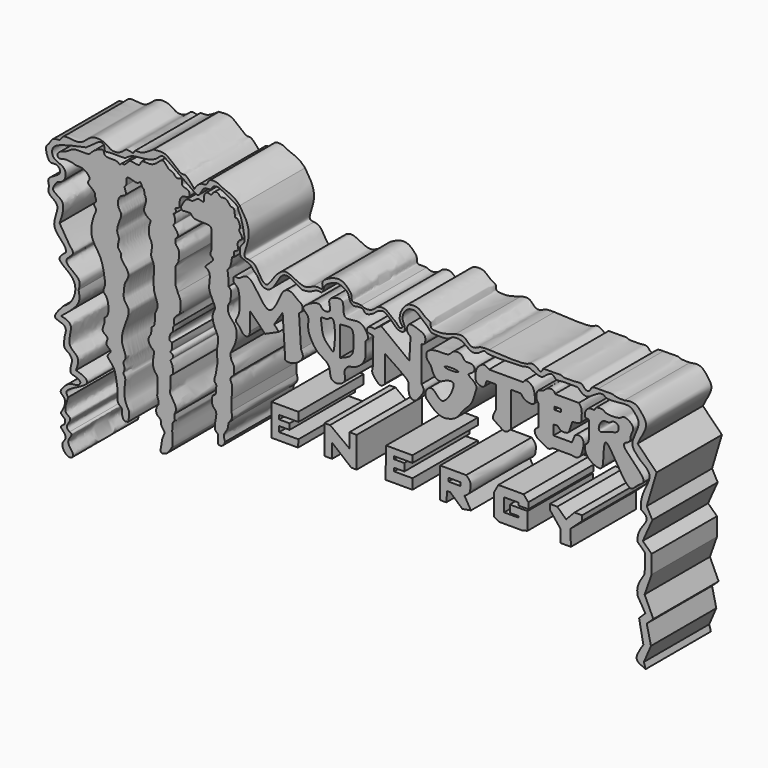
from build123d import *

# Parameters (mm, degrees)
F3_DEPTH = 25
F2_W     = 3.7656910717
F2_H     = 1.0270066559
F2_W_2   = 2.1294355392
F2_H_2   = 0.8966038004


# Not quite as in the source:
# - the program builds the solid bodies; features that only make, move or delete a surface that nothing else refers to are left out


with BuildPart() as f3:
    # F2 (on Front) → F3 (new body)
    with BuildSketch(Plane.XZ):
        Polygon((-21.8279026449, -32.0507697761), (-13.6387161911, -32.0507697761), (-13.5350553319, -29.7702345997), (-19.4437094033, -29.7702345997), (-19.4437094033, -28.1116645783), (-16.230231151, -28.1116645783), (-16.230231151, -26.3494346291), (-19.4437094033, -26.3494346291), (-19.4437094033, -25.1055080444), (-13.5350553319, -25.1055080444), (-13.5350553319, -22.3585031927), (-21.8279026449, -22.3585031927), align=None)
    extrude(amount=F3_DEPTH)


with BuildPart() as f3b:
    # F2 (on Front) → F3, piece 2 (new body)
    with BuildSketch(Plane.XZ):
        Polygon((-3.8289250806, -22.7761287242), (-5.5911550298, -22.8279586881), (-5.5911550298, -31.6909402609), (-3.2069615554, -31.6909402609), (-3.2069615554, -27.3371953517), (2.6498620864, -32.1574136615), (4.3084332719, -32.1574136615), (4.3084332719, -22.7761287242), (2.079728758, -22.7761287242), (2.079728758, -27.1817035973), align=None)
    extrude(amount=F3_DEPTH)


with BuildPart() as f3c:
    # F2 (on Front) → F3, piece 3 (new body)
    with BuildSketch(Plane.XZ):
        Polygon((21.3820878416, -22.7204784751), (13.3220171556, -22.7204784751), (13.1144626066, -32.0258811116), (21.3820878416, -32.0258811116), (21.3820878416, -28.9125498384), (15.7780908048, -28.9125498384), (15.7780908048, -27.909366414), (18.891422078, -27.909366414), (18.891422078, -25.6262551993), (15.7089047134, -25.6262551993), (15.7089047134, -24.7960332781), (21.3820878416, -24.7960332781), align=None)
    extrude(amount=F3_DEPTH)


with BuildPart() as f3d:
    # F2 (on Front) → F3, piece 4 (new body)
    with BuildSketch(Plane.XZ):
        with BuildLine():
            Line((29.8660583794, -32.0507697761), (31.7277424037, -32.0507697761))
            Line((31.7277424037, -32.0507697761), (32.0186279714, -28.9156045765))
            Line((32.0186279714, -28.9156045765), (32.9494699836, -28.9156045765))
            Line((32.9494699836, -28.9156045765), (36.6728305817, -32.2317257524))
            Line((36.6728305817, -32.2317257524), (39.2908193171, -31.7663066089))
            Line((39.2908193171, -31.7663066089), (37.3127833009, -28.450185433))
            add(Edge.make_bspline(
                [(37.8363840282, -22.7204784751), (38.3456048869, -23.1865278474), (39.3238666476, -24.0818530718), (39.1050914631, -25.8334312431), (38.977892404, -27.3696127917), (37.8928678318, -28.0737395457), (37.3127833009, -28.450185433)],
                knots=[0, 0, 0, 0, 0.2644850367, 0.5081009414, 0.7370169838, 1, 1, 1, 1], degree=3))
            Line((37.8363840282, -22.7204784751), (29.8660583794, -22.7204784751))
            Line((29.8660583794, -22.7204784751), (29.8660583794, -32.0507697761))
        make_face()
        with Locations((34.2598091811, -25.7162433118)):
            Rectangle(F2_W, F2_H, mode=Mode.SUBTRACT)
    extrude(amount=F3_DEPTH)


with BuildPart() as f3e:
    # F2 (on Front) → F3, piece 5 (new body)
    with BuildSketch(Plane.XZ):
        Polygon((47.8596165776, -32.0507697761), (55.1240593195, -32.0507697761), (56.6234141588, -31.6276736557), (56.6234141588, -26.305552572), (51.1786416173, -26.305552572), (51.1786416173, -28.5543948412), (53.8787283003, -28.5543948412), (53.8787283003, -28.990233317), (49.4352839887, -28.990233317), (49.4352839887, -24.9151382595), (53.8787283003, -24.9151382595), (53.8787283003, -25.7161445916), (56.8536892533, -25.7161445916), (56.8536892533, -23.8481462002), (55.4007999599, -22.1633397041), (47.6769925559, -22.1633397041), (46.4067310095, -24.4708117098), (46.4067310095, -31.2509573996), align=None)
    extrude(amount=F3_DEPTH)


with BuildPart() as f3f:
    # F2 (on Front) → F3, piece 6 (new body)
    with BuildSketch(Plane.XZ):
        Polygon((66.6389763355, -31.6276736557), (69.8906779289, -31.6276736557), (69.7407498956, -26.8117766827), (73.2039138675, -23.625664413), (73.3251263795, -22.0095198601), (70.9874853492, -22.0095198601), (68.4235452277, -24.7108214691), (65.7234713435, -22.1480466425), (63.4608715773, -22.1480466425), (63.4608715773, -23.7180143595), (66.6389763355, -27.7352873236), align=None)
    extrude(amount=F3_DEPTH)


with BuildPart() as f3g:
    # F2 (on Front) → F3, piece 7 (new body)
    with BuildSketch(Plane.XZ):
        with BuildLine():
            add(Edge.make_bspline(
                [(3.503452288, -4.7838860191), (2.8113226503, -5.0136695081), (1.7830241675, -4.8630734081), (0.0911722194, -6.7811448987), (1.3671495093, -9.3955288011), (-1.4418505197, -11.2815872593), (-4.1217897443, -10.3505317517), (-3.5555284745, -6.4965573266), (-7.1381809371, -4.9981730676), (-9.1052398705, -2.8089888848), (-11.0325887604, 0.9634765262), (-10.0411178915, 4.3471198689), (-11.9148876299, 5.5223323903), (-12.4373031281, 6.7516798684), (-6.8099838065, 9.8665488087), (-6.462441494, 7.1877744687), (-2.9120184289, 7.5155698662), (-5.0031559191, 11.1051679105), (-1.8479274649, 12.3233814583), (0.6824877872, 12.1855257293), (-0.2774898152, 7.0730316824), (3.5047921516, 7.8935101918), (6.0050121897, 7.9486113123), (7.6235614634, 5.625519934), (7.9974005866, 3.995709803), (6.4584911773, 3.5935713271), (8.0066750098, -1.999760349), (4.6370015267, -4.4075534873), (3.503452288, -4.7838860191)],
                knots=[0, 0, 0, 0, 0.0315220967, 0.0654446519, 0.1026152705, 0.1419423819, 0.1771472788, 0.2195443707, 0.263519259, 0.3050564981, 0.3533625845, 0.3957388119, 0.4280430375, 0.4505910626, 0.5046572349, 0.5359398579, 0.5707371212, 0.6103314602, 0.6494294844, 0.6822119863, 0.7277784762, 0.7674991504, 0.8053447517, 0.8441561314, 0.8719949007, 0.8952996773, 0.9483740519, 1, 1, 1, 1], degree=3))
        make_face()
        with BuildLine():
            add(Edge.make_bspline(
                [(-3.3008460887, -2.4911721703), (-3.7924419075, -2.0137396744), (-5.5897346622, -0.5109165894), (-6.3523235923, 1.7697391653), (-6.4166270756, 3.9327068913), (-6.9610982752, 5.752738943), (-4.5225481233, 5.2057664601), (-4.252961633, 5.9994852498), (-1.8495900551, 7.0522733141), (-2.4371710556, -3.4390093796), (-3.1018362507, -2.6844483537), (-3.3008460887, -2.4911721703)],
                knots=[0, 0, 0, 0, 0.1325905556, 0.2546628881, 0.3725255143, 0.4599015989, 0.5640922214, 0.6328553126, 0.7173438444, 0.9463241468, 1, 1, 1, 1], degree=3))
        make_face(mode=Mode.SUBTRACT)
        with BuildLine():
            Line((-0.8801673539, -3.7418559659), (-0.8801673539, 5.3356890567))
            add(Edge.make_bspline(
                [(-0.8801673539, -3.7418559659), (0.1051218784, -3.3629410883), (1.8893722855, -2.6767679297), (3.4229442665, -1.1878230291), (3.2897460639, 2.5173382681), (3.3267032878, 4.3339201727), (2.7130035187, 5.6249956516), (0.9045163806, 5.5591126678), (-0.2714937046, 5.4118885883), (-0.8801673539, 5.3356890567)],
                knots=[0, 0, 0, 0, 0.1705659116, 0.3088761019, 0.495841013, 0.6324582839, 0.7383649585, 0.8645841924, 1, 1, 1, 1], degree=3))
        make_face(mode=Mode.SUBTRACT)
    extrude(amount=F3_DEPTH)


with BuildPart() as f3h:
    # F2 (on Front) → F3, piece 8 (new body)
    with BuildSketch(Plane.XZ):
        with BuildLine():
            Line((13.0070131272, -6.1348984018), (13.0070131272, 1.909989398))
            add(Edge.make_bspline(
                [(24.1350065917, -2.6675420813), (24.4988556117, -3.1186405426), (25.3127079876, -4.1276512428), (23.650589719, -6.2059967045), (22.2456584652, -8.257711553), (19.9145445459, -7.0406724044), (20.3702129266, -3.7004981152), (19.5456257752, -2.444477126), (15.7190605129, 0.103869325), (13.0070131272, 1.909989398)],
                knots=[0, 0, 0, 0, 0.1108514285, 0.2479509179, 0.379166634, 0.4977873803, 0.650360402, 0.752195744, 1, 1, 1, 1], degree=3))
            Line((24.1350065917, -2.6675420813), (24.1350065917, 8.1594744697))
            add(Edge.make_bspline(
                [(20.7801572978, 9.0236030519), (20.3457138528, 9.3864533714), (19.4836634842, 10.1064440978), (19.8580530262, 11.8427016223), (20.7640873111, 12.7051879525), (23.6254897157, 11.6752187346), (25.5643978554, 10.8490187459), (25.2435917704, 8.2790753792), (24.4553801465, 8.1940383167), (24.1350065917, 8.1594744697)],
                knots=[0, 0, 0, 0, 0.1400032029, 0.2778032769, 0.3898219931, 0.5785225018, 0.7357644761, 0.8925998151, 1, 1, 1, 1], degree=3))
            Line((20.7801572978, 9.0236030519), (20.4243399203, 2.4155643769))
            Line((20.4243399203, 2.4155643769), (11.7830587551, 9.0236030519))
            Line((11.7830587551, 9.0236030519), (9.7907502204, 7.5596827082))
            add(Edge.make_bspline(
                [(9.319582954, 4.8124021851), (9.3803734347, 5.0462029175), (9.5213533732, 5.5884130216), (8.2738494629, 5.8541952014), (7.31455102, 5.9431960106), (7.6227500043, 7.9209294321), (9.0216714014, 7.6878317747), (9.7907502204, 7.5596827082)],
                knots=[0, 0, 0, 0, 0.1505740167, 0.3491980219, 0.518685682, 0.7353899597, 1, 1, 1, 1], degree=3))
            Line((9.319582954, 4.8124021851), (9.319582954, -2.5581021328))
            add(Edge.make_bspline(
                [(13.0070131272, -6.1348984018), (12.6049051159, -6.6177685747), (11.7230780125, -7.6767079492), (9.7804141481, -5.6927668504), (8.8350286003, -4.3052662439), (9.1578579839, -3.1412360196), (9.319582954, -2.5581021328)],
                knots=[0, 0, 0, 0, 0.2356288847, 0.5167366256, 0.7579038379, 1, 1, 1, 1], degree=3))
        make_face()
    extrude(amount=F3_DEPTH)


with BuildPart() as f3i:
    # F2 (on Front) → F3, piece 9 (new body)
    with BuildSketch(Plane.XZ):
        with BuildLine():
            add(Edge.make_bspline(
                [(25.5756434053, -6.0040308163), (25.4061184127, -5.3832063219), (25.0512461325, -4.0836138516), (27.7019975714, -1.5243889893), (30.5978060983, -8.0140858299), (35.5163682682, 1.9393601204), (32.6292719516, 1.0476557915), (31.5465591848, 0.7132507162)],
                knots=[0, 0, 0, 0, 0.1540710504, 0.3225220314, 0.5423303079, 0.8283656781, 1, 1, 1, 1], degree=3))
            add(Edge.make_bspline(
                [(31.5465591848, 0.7132507162), (30.7752444483, 0.2979041147), (29.2896538825, -0.502074109), (27.5616896872, 1.2528426912), (27.2311493936, 3.3454250283), (25.4632454929, 4.7198831161), (25.630185434, 6.9245563777), (27.5651484443, 7.7095666937), (29.4398172278, 7.9487657515), (32.7819511773, 7.6664383296), (33.6271863146, 9.6029162043), (36.6279698804, 9.746479837), (37.2599515094, 7.3287532722), (40.1594276723, 8.2934727633), (40.710330294, 5.6568483335), (37.744488116, 4.7230480927), (39.8729507504, 3.6633294807), (41.281821717, 2.1909886005), (40.6500063641, 0.6727985282), (40.1459108495, -1.2832116041), (39.1348857054, -3.6137690615), (36.8162707519, -5.277491669), (35.2307491259, -8.3624235277), (32.852026237, -9.2006117011), (30.7539983625, -9.7184551513), (28.1525717486, -8.6347645017), (26.4838434223, -6.9311937248), (25.5756434053, -6.0040308163)],
                knots=[0, 0, 0, 0, 0.0412451727, 0.0794402551, 0.1184972014, 0.1573515408, 0.1934023274, 0.2298199639, 0.2684388174, 0.3152434581, 0.351665482, 0.393139999, 0.4303795974, 0.4708563309, 0.5060832175, 0.5447731774, 0.577939634, 0.6159501126, 0.6481405375, 0.6867402637, 0.7290134368, 0.7744765682, 0.8237433298, 0.8654243276, 0.9041083893, 0.9478112997, 1, 1, 1, 1], degree=3))
        make_face()
        with BuildLine():
            add(Edge.make_bspline(
                [(31.1507247388, 4.3506226502), (31.1507247388, 3.7075211871), (34.3530811369, 4.0290719187), (37.555437535, 4.3506226502), (34.3530811369, 4.6721733818), (31.1507247388, 4.9937241134), (31.1507247388, 4.3506226502)],
                knots=[0, 0, 0, 2.0943951024, 2.0943951024, 4.1887902048, 4.1887902048, 6.2831853072, 6.2831853072, 6.2831853072], degree=2, weights=[1, 0.5, 1, 0.5, 1, 0.5, 1]))
        make_face(mode=Mode.SUBTRACT)
    extrude(amount=F3_DEPTH)


with BuildPart() as f3j:
    # F2 (on Front) → F3, piece 10 (new body)
    with BuildSketch(Plane.XZ):
        with BuildLine():
            add(Edge.make_bspline(
                [(46.1458899081, -3.782347776), (46.0621870803, -4.1873362767), (45.8738035332, -5.0988128932), (47.6676565444, -5.7970314374), (49.7249420098, -7.7386388048), (50.9412470515, -6.4798566337), (51.5339821577, -5.8664213866)],
                knots=[0, 0, 0, 0, 0.194995116, 0.4388605805, 0.7265430776, 1, 1, 1, 1], degree=3))
            Line((51.5339821577, -5.8664213866), (51.5339821577, 4.7572711483))
            Line((51.5339821577, 4.7572711483), (54.5838475227, 4.7572711483))
            add(Edge.make_bspline(
                [(54.5838475227, 4.7572711483), (54.9445359485, 4.2186451045), (55.7106902411, 3.0745256205), (59.1133915488, 2.6685733866), (58.8718377024, 5.3408831184), (58.5497843618, 7.3499903122), (57.6343725322, 8.294083257), (56.0271563643, 9.1028773107), (55.4934462233, 8.3577911301), (55.2446506917, 8.0104600638)],
                knots=[0, 0, 0, 0, 0.1520231156, 0.3229190466, 0.4765642291, 0.6312552419, 0.7532387675, 0.8849692234, 1, 1, 1, 1], degree=3))
            Line((55.2446506917, 8.0104600638), (44.8242835701, 8.0104600638))
            add(Edge.make_bspline(
                [(44.8242835701, 8.0104600638), (44.3675333804, 8.3812585434), (43.4351991209, 9.1381452043), (41.7182434822, 8.0942774619), (40.7928768985, 6.715734308), (40.7244007336, 5.503812826), (40.5013842137, 3.5345446953), (41.9256017521, 2.7331848104), (43.5124763065, 2.5734174703), (43.8654087108, 3.9438101521), (44.0618172288, 4.7064400278)],
                knots=[0, 0, 0, 0, 0.1263456942, 0.257901194, 0.3839642943, 0.4945421325, 0.6272741385, 0.7471622588, 0.8592946258, 1, 1, 1, 1], degree=3))
            Line((44.0618172288, 4.7064400278), (46.9083562493, 4.7064400278))
            Line((46.9083562493, 4.7064400278), (46.9083562493, -2.1049224306))
            Line((46.9083562493, -2.1049224306), (46.1458899081, -3.782347776))
        make_face()
    extrude(amount=F3_DEPTH)


with BuildPart() as f3k:
    # F2 (on Front) → F3, piece 11 (new body)
    with BuildSketch(Plane.XZ):
        with BuildLine():
            Line((60.0227750838, 3.7914810237), (60.0227750838, -2.6132331695))
            add(Edge.make_bspline(
                [(64.3434152007, -6.832211744), (63.8654350673, -7.1179865312), (62.9326108336, -7.675703533), (61.7600801197, -6.7056123664), (59.3215288239, -5.836178243), (58.4373942726, -3.5871466736), (59.508556375, -2.9291222865), (60.0227750838, -2.6132331695)],
                knots=[0, 0, 0, 0, 0.1834163448, 0.3579546498, 0.600798013, 0.8083603501, 1, 1, 1, 1], degree=3))
            Line((64.3434152007, -6.832211744), (70.1889842749, -6.832211744))
            add(Edge.make_bspline(
                [(70.1889842749, -3.375699278), (70.4148223508, -2.8932615015), (70.8323825076, -2.0012649115), (71.1257228135, -0.7286505648), (73.4044397159, -0.739241943), (73.9493742107, -2.6496728362), (73.3359252152, -5.0612214192), (72.8357815171, -6.2298458673), (71.7438159103, -7.2284700423), (70.7231798895, -6.9683547452), (70.1889842749, -6.832211744)],
                knots=[0, 0, 0, 0, 0.1244118259, 0.2300295081, 0.3614939824, 0.4921845047, 0.6497085426, 0.763524384, 0.8762298856, 1, 1, 1, 1], degree=3))
            Line((70.1889842749, -3.375699278), (64.5467340946, -3.375699278))
            Line((64.5467340946, -3.375699278), (64.5467340946, -0.4274974926))
            add(Edge.make_bspline(
                [(72.3238885403, 7.9596284777), (72.63021509, 7.5811847571), (73.3173005105, 6.7323417067), (73.1676826384, 4.4498725395), (73.1524790454, 2.2965562825), (70.6013324969, 2.3127340198), (70.1300932481, 2.1354405001), (69.487877771, -0.896432615), (68.5601900748, -1.4358394608), (66.5066609501, -1.4827146567), (65.9532404189, -0.1015352018), (65.0209514532, -0.3175961194), (64.5467340946, -0.4274974926)],
                knots=[0, 0, 0, 0, 0.097480458, 0.2186470665, 0.3261227099, 0.4414283747, 0.4968792825, 0.6319473283, 0.7154650187, 0.8224668493, 0.9096961298, 1, 1, 1, 1], degree=3))
            Line((72.3238885403, 7.9596284777), (65.0042146444, 7.9596284777))
            add(Edge.make_bspline(
                [(60.0227750838, 3.7914810237), (59.805578228, 4.0200896126), (59.3009055391, 4.5512782932), (59.2927331203, 6.3458639995), (59.883365164, 7.5765765519), (61.5230093611, 7.4517061115), (62.5456824427, 9.0597869776), (64.7233814002, 9.0194713975), (64.9211472045, 8.2731185644), (65.0042146444, 7.9596284777)],
                knots=[0, 0, 0, 0, 0.1211424616, 0.2814833189, 0.414256649, 0.5569143261, 0.7195607436, 0.8822072847, 1, 1, 1, 1], degree=3))
        make_face()
        with Locations((65.8582672477, 4.1072387248)):
            Rectangle(F2_W_2, F2_H_2, mode=Mode.SUBTRACT)
    extrude(amount=F3_DEPTH)


with BuildPart() as f3l:
    # F2 (on Front) → F3, piece 12 (new body)
    with BuildSketch(Plane.XZ):
        with BuildLine():
            add(Edge.make_bspline(
                [(75.4084140062, 3.9207721129), (75.3741883861, 4.3777174645), (75.3148136264, 4.7525146004), (74.2224928646, 4.2153509758), (73.970151299, 6.4596143139), (75.6958439244, 7.9144692863), (77.2720321691, 7.3432219286), (77.1761140426, 8.6606724241), (80.0304182882, 8.6772390387), (80.2092108361, 7.7101246036), (85.0612902981, 7.4997966152), (86.0465785249, 9.2819059317), (89.8548287118, 6.9104373811), (87.9546387233, 4.51968954), (88.2759913555, 2.3848233183), (86.1874151654, 1.9301512263), (85.7199509041, 0.0324046881), (94.3313008747, -6.8338335231), (90.0323028023, -8.0345776864), (87.4212655088, -12.7029106449), (79.3644786325, 5.8849768065), (80.1559883718, -6.3609431851), (78.8381409115, -8.0543767975), (75.8276242824, -6.7297178446), (74.1032864345, -4.775439151), (74.1069814932, -2.2396911603), (75.6958464037, -2.3665177055), (75.5070732487, 2.6035751686), (75.4084140062, 3.9207721129)],
                knots=[0, 0, 0, 0, 0.0203919358, 0.0405098051, 0.0718152932, 0.1069671347, 0.133818873, 0.1552581713, 0.1920879182, 0.2144793905, 0.2646315633, 0.2965564759, 0.3397576718, 0.3779602749, 0.4109993651, 0.4422343123, 0.4706853247, 0.5437035151, 0.5831431777, 0.6247365762, 0.7090619367, 0.7690785607, 0.8026792394, 0.8432780935, 0.8835139261, 0.9176211952, 0.9412179259, 1, 1, 1, 1], degree=3))
        make_face()
        with BuildLine():
            add(Edge.make_bspline(
                [(78.5704776645, 2.5322814472), (78.126093586, 3.0403921697), (79.1692033775, 6.2339507213), (81.766742196, 5.2935144941), (82.5171446118, 6.6457313561), (84.3630740041, 6.1527962778), (84.6267575644, 5.0552225028), (84.101615557, 3.5761658857), (81.972310774, 3.5074956738), (79.0429563472, 1.9920472298), (78.5704776645, 2.5322814472)],
                knots=[0, 0, 0, 0, 0.1570021124, 0.2909462665, 0.3910850546, 0.5038714922, 0.594944461, 0.6964936405, 0.8330719869, 1, 1, 1, 1], degree=3))
        make_face(mode=Mode.SUBTRACT)
    extrude(amount=F3_DEPTH)


with BuildPart() as f3m:
    # F2 (on Front) → F3, piece 13 (new body)
    with BuildSketch(Plane.XZ):
        with BuildLine():
            add(Edge.make_bspline(
                [(-32.3238708079, 5.2692117169), (-32.1339182853, 4.9733019987), (-31.5376614734, 4.0444478679), (-31.2397648639, -2.4563880266), (-33.3374242305, -4.0470383654), (-31.2234373463, -5.3677292796), (-30.7515536056, -7.133049429), (-28.600863174, -7.4064643528), (-28.4359431494, -6.1008449236), (-28.3504724503, -5.4242005572)],
                knots=[0, 0, 0, 0, 0.1138197558, 0.3572777229, 0.4918572745, 0.623719343, 0.7536919969, 0.8723495385, 1, 1, 1, 1], degree=3))
            Line((-28.3504724503, -5.4242005572), (-28.3504724503, 0))
            Line((-28.3504724503, 0), (-23.736583069, -4.6778358519))
            Line((-23.736583069, -4.6778358519), (-19.5297989994, -2.7779988013))
            Line((-19.5297989994, -2.7779988013), (-20.9546778351, -1.2174181174))
            Line((-20.9546778351, -1.2174181174), (-18.3763280511, 2.7858105022))
            Line((-18.3763280511, 2.7858105022), (-17.562109977, -9.8345372826))
            add(Edge.make_bspline(
                [(-17.562109977, -9.8345372826), (-16.8573217322, -9.9726467263), (-15.2462265037, -10.2883549796), (-11.5049291375, -7.6449185626), (-12.3701357237, -6.0003849647), (-12.7446670085, -5.2884980105)],
                knots=[0, 0, 0, 0, 0.3060468226, 0.699601021, 1, 1, 1, 1], degree=3))
            Line((-12.7446670085, -5.2884980105), (-13.3553287014, 4.2785396799))
            add(Edge.make_bspline(
                [(-13.3553287014, 4.2785396799), (-12.9174906886, 4.610595199), (-12.0622469873, 5.2592104011), (-12.3204340314, 7.0157312244), (-13.6896025156, 7.5548883564), (-15.6449235352, 9.517252599), (-17.6597215061, 9.2711170922), (-19.0272382675, 7.6031334106), (-22.6810409105, -2.2649330056), (-28.3073016542, 11.5616524723), (-31.6899586493, 7.078625447), (-33.2209086153, 8.2469751914), (-33.7508681695, 6.2768813441), (-32.8181286633, 5.6182303222), (-32.3238708079, 5.2692117169)],
                knots=[0, 0, 0, 0, 0.0655583558, 0.128057339, 0.1909733128, 0.2771894171, 0.3446587121, 0.4265714586, 0.5593874834, 0.7185611162, 0.8130760838, 0.8711607475, 0.9317281918, 1, 1, 1, 1], degree=3))
        make_face()
    extrude(amount=F3_DEPTH)


with BuildPart() as f3n:
    # F2 (on Front) → F3, piece 14 (new body)
    with BuildSketch(Plane.XZ):
        with BuildLine():
            add(Edge.make_bspline(
                [(86.277499795, 13.1921237335), (87.4185934495, 13.4133239742), (89.7041230289, 13.8563723525), (91.9428358923, 11.0326804296), (93.618626085, 8.5033308377), (91.0277669662, 4.4446822814), (90.5058294107, 3.2887497817), (90.3034508228, 2.840542933)],
                knots=[0, 0, 0, 0, 0.2067961155, 0.4141979382, 0.6057598121, 0.847135406, 1, 1, 1, 1], degree=3))
            add(Edge.make_bspline(
                [(78.1892538071, 13.6597929522), (79.0037100185, 13.6430028032), (80.5555373353, 13.6110116272), (82.7083507687, 13.8119139889), (83.57934085, 13.1749481923), (85.2416850518, 13.1855300972), (86.277499795, 13.1921237335)],
                knots=[0, 0, 0, 0, 0.2791933404, 0.5319621192, 0.7083633241, 1, 1, 1, 1], degree=3))
            add(Edge.make_bspline(
                [(61.4448413253, 13.6597929522), (62.8836419565, 13.6341922981), (65.222990656, 13.5925681455), (66.8907976686, 13.8037138262), (67.7929704204, 13.178266488), (69.5864513165, 13.4100423778), (71.0638150635, 13.2149328766), (73.3381001728, 13.7833015954), (74.1674849758, 11.9407678044), (75.8559700127, 12.0542656014), (75.9632479753, 13.7064292897), (77.387818533, 13.6765835668), (78.1892538071, 13.6597929522)],
                knots=[0, 0, 0, 0, 0.150835137, 0.2452431379, 0.3208180625, 0.4200706757, 0.5169310526, 0.6252244461, 0.72420674, 0.8081835775, 0.8920878672, 1, 1, 1, 1], degree=3))
            add(Edge.make_bspline(
                [(44.8618084192, 13.3370347321), (49.7544030227, 13.0701222135), (56.3442876354, 12.7106150722), (57.5958501654, 14.1214390329), (59.4911622048, 13.5156787161), (60.5950899585, 12.1392879899), (61.1605113114, 13.1510262542), (61.4448413253, 13.6597929522)],
                knots=[0, 0, 0, 0, 0.4126534402, 0.5558070464, 0.717317611, 0.8578492178, 1, 1, 1, 1], degree=3))
            add(Edge.make_bspline(
                [(34.6134118736, 14.2649617046), (35.5407104435, 14.4521960002), (37.3889430992, 14.8253795146), (38.8831583693, 12.194111617), (40.9995006141, 12.500427315), (42.1181380365, 13.3862405962), (43.8500857494, 13.3551792908), (44.8618084192, 13.3370347321)],
                knots=[0, 0, 0, 0, 0.2185605916, 0.4356210995, 0.6168416239, 0.776176837, 1, 1, 1, 1], degree=3))
            add(Edge.make_bspline(
                [(17.8286470473, 14.8297864944), (18.2466753756, 15.5681988492), (19.0174317192, 16.9296759743), (20.5773984068, 17.761344641), (22.8327722921, 17.7606640336), (24.0173706321, 16.9921167848), (25.639540267, 15.3998181248), (27.1770300194, 15.0886197574), (26.7182995679, 13.1571311059), (28.7278853969, 13.1000844501), (30.2049910369, 13.0008951024), (32.5628763782, 13.5486912834), (33.9370823417, 14.0287137393), (34.6134118736, 14.2649617046)],
                knots=[0, 0, 0, 0, 0.1041266733, 0.1919876921, 0.2896821544, 0.3702369986, 0.4715670528, 0.5483807885, 0.62683907, 0.710712182, 0.7963958974, 0.8997941567, 1, 1, 1, 1], degree=3))
            add(Edge.make_bspline(
                [(5.7242442854, 12.6108312979), (6.1674645712, 12.3924054039), (7.1362961312, 11.9149500472), (9.4535655573, 12.4217412056), (10.466766911, 13.9110660271), (13.0516062461, 14.3665970707), (14.7816187647, 12.5111230257), (16.5523417101, 11.4869723661), (17.4842861913, 9.9925437502), (18.6891040586, 10.9455037796), (17.1151582194, 12.2103740762), (17.5695842917, 13.8786963404), (17.8286470473, 14.8297864944)],
                knots=[0, 0, 0, 0, 0.0916701362, 0.2003809931, 0.2984337676, 0.4092400816, 0.524162285, 0.6329193316, 0.7215433956, 0.7891094781, 0.8797738883, 1, 1, 1, 1], degree=3))
            add(Edge.make_bspline(
                [(-5.4521509446, 15.91909118), (-4.5944789682, 16.407901969), (-2.9016691373, 17.3726807328), (0.1156349158, 17.5562559472), (2.0108324857, 15.4802790804), (2.8827745247, 14.5105554131), (2.5936645035, 12.497536046), (4.2830744099, 12.7616892988), (5.2283697286, 12.6627381866), (5.7242442854, 12.6108312979)],
                knots=[0, 0, 0, 0, 0.1760878818, 0.3475493028, 0.5132391692, 0.6312584364, 0.7575044304, 0.8727938447, 1, 1, 1, 1], degree=3))
            add(Edge.make_bspline(
                [(-9.1641684994, 12.8528987989), (-8.5133667974, 13.0294458386), (-7.4004240907, 13.3313607531), (-5.9455298962, 12.7764600753), (-6.4993905865, 14.9305290032), (-5.7934890115, 15.5968784896), (-5.4521509446, 15.91909118)],
                knots=[0, 0, 0, 0, 0.2877611679, 0.4921033428, 0.7544070316, 1, 1, 1, 1], degree=3))
            add(Edge.make_bspline(
                [(-28.7329517305, 13.7001359835), (-28.2005918727, 13.5857994872), (-27.0356354654, 13.3355983646), (-25.9113392201, 11.5927665179), (-23.5452468608, 7.2520058428), (-21.1880186629, 11.3837602909), (-19.5554295124, 13.2092978283), (-17.0313876159, 14.8949127844), (-12.1764019432, 11.2257819055), (-10.072445388, 12.3622752477), (-9.1641684994, 12.8528987989)],
                knots=[0, 0, 0, 0, 0.0912905214, 0.1997699044, 0.3372534416, 0.4695341734, 0.5902790758, 0.7042892825, 0.8723418458, 1, 1, 1, 1], degree=3))
            add(Edge.make_bspline(
                [(-31.5169654787, 27.3767374456), (-30.6347738533, 26.0504254662), (-28.9692410928, 23.5464161459), (-28.548207452, 19.7794551217), (-29.6492208491, 16.4713809377), (-30.4209886324, 13.8476082473), (-29.2460535878, 13.744962191), (-28.7329517305, 13.7001359835)],
                knots=[0, 0, 0, 0, 0.2501647138, 0.4722982109, 0.6957055162, 0.8671125987, 1, 1, 1, 1], degree=3))
            add(Edge.make_bspline(
                [(-45.4278662801, 27.3767374456), (-44.7455452058, 28.2891152968), (-43.575596155, 29.8535336346), (-41.5272690271, 29.2256253529), (-41.1582369479, 31.6987441976), (-37.9610392989, 31.3836973061), (-36.5075379003, 30.1804216633), (-33.5845567645, 29.4928292429), (-32.2111285799, 28.0871838741), (-31.5169654787, 27.3767374456)],
                knots=[0, 0, 0, 0, 0.1607139781, 0.2755699233, 0.399764796, 0.5510490082, 0.682627519, 0.8395924387, 1, 1, 1, 1], degree=3))
            add(Edge.make_bspline(
                [(-57.6108247042, 33.9393392205), (-56.5904608095, 34.0317161297), (-54.6020889506, 34.2117299928), (-52.6009130719, 32.8040721674), (-49.3390235075, 29.7568605887), (-48.0968047106, 30.5890837949), (-46.4960686851, 28.6624306848), (-45.4278662801, 27.3767374456)],
                knots=[0, 0, 0, 0, 0.2038137466, 0.3971695984, 0.6408815078, 0.7603532182, 1, 1, 1, 1], degree=3))
            Line((-57.6108247042, 33.9393392205), (-57.9158291221, 33.9393392205))
            add(Edge.make_bspline(
                [(-90.6876251101, 22.3766118288), (-90.782291049, 23.0372911855), (-90.9599331736, 24.2770664003), (-89.6705222414, 25.0788583124), (-88.8857289778, 27.2756676653), (-86.2343320891, 26.7399517192), (-85.7861011249, 29.3767483168), (-80.0258318392, 27.3990779288), (-77.4283141736, 31.6139831739), (-72.9859558884, 31.320598114), (-71.2519637243, 29.6017208165), (-69.3182030396, 29.2886407843), (-67.3111525741, 30.1369378152), (-66.2552699779, 31.6713401771), (-63.8270188941, 30.5372765992), (-63.8085741699, 32.0678548219), (-61.5908061278, 31.3989654138), (-59.3245945596, 32.9655124968), (-57.9158291221, 33.9393392205)],
                knots=[0, 0, 0, 0, 0.0549771793, 0.1031655426, 0.1617489747, 0.2209866699, 0.2747506822, 0.3651386797, 0.4513471014, 0.5321937992, 0.595383924, 0.6507211979, 0.7103087922, 0.7635282229, 0.8215405324, 0.8584134717, 0.9119842956, 1, 1, 1, 1], degree=3))
            add(Edge.make_bspline(
                [(-89.8913815618, 13.7024139985), (-90.1036135358, 14.4340407961), (-90.5956789092, 16.13033663), (-86.5927448955, 17.4071703301), (-86.3363595804, 19.2937374018), (-87.8103325705, 20.4965731215), (-89.789936789, 19.7037633438), (-90.3684921841, 21.4264001151), (-90.6876251101, 22.3766118288)],
                knots=[0, 0, 0, 0, 0.1658141707, 0.3844444843, 0.5251281736, 0.6703029437, 0.818138095, 1, 1, 1, 1], degree=3))
            add(Edge.make_bspline(
                [(-84.6553444862, -2.5635273196), (-84.7048596724, -2.0234137759), (-84.8391958784, -0.5580693061), (-90.0587733282, 3.1780521509), (-85.7664354392, 9.5665359131), (-90.4395412989, 11.223007773), (-90.0596671517, 12.9412337968), (-89.8913815618, 13.7024139985)],
                knots=[0, 0, 0, 0, 0.1442109757, 0.3912487627, 0.6468882864, 0.8435702628, 1, 1, 1, 1], degree=3))
            add(Edge.make_bspline(
                [(-85.6432646293, -17.3617769033), (-84.640812152, -16.7386259806), (-82.3973201361, -15.3440121198), (-80.7660392644, -8.6272468225), (-88.380958138, -5.3269386044), (-85.7611771262, -3.3837600872), (-84.6553444862, -2.5635273196)],
                knots=[0, 0, 0, 0, 0.2253559688, 0.5043474161, 0.7907806787, 1, 1, 1, 1], degree=3))
            add(Edge.make_bspline(
                [(-85.1055532694, -25.3500156105), (-84.8019723687, -24.2727921813), (-84.1791842662, -22.0628971131), (-88.3775031021, -21.6379352764), (-87.9176893485, -19.9221125606), (-86.5326229502, -18.3629337242), (-85.6432646293, -17.3617769033)],
                knots=[0, 0, 0, 0, 0.2620516411, 0.5375919365, 0.7030853831, 1, 1, 1, 1], degree=3))
            add(Edge.make_bspline(
                [(-86.2191617489, -39.9951227009), (-85.3984315809, -38.9970476091), (-83.8781977707, -37.1483188076), (-81.0374016676, -37.4879838948), (-79.8678095906, -35.9588191513), (-81.6213862848, -35.0056317568), (-83.6178058901, -34.8642876167), (-83.1822126173, -32.3905150144), (-82.5711453354, -30.8488503773), (-83.9200726999, -29.1008277364), (-85.5441259678, -28.6343154789), (-85.2697452947, -26.5795856428), (-85.1055532694, -25.3500156105)],
                knots=[0, 0, 0, 0, 0.1328376608, 0.2460544417, 0.324546787, 0.4136906629, 0.5051090366, 0.6051167978, 0.6961496275, 0.7939780851, 0.8767145111, 1, 1, 1, 1], degree=3))
            add(Edge.make_bspline(
                [(-85.1055532694, -48.9613488317), (-84.9802364741, -48.476268915), (-84.71941225, -47.4666628791), (-86.7432409936, -46.4458491259), (-85.4221051871, -45.2152748196), (-84.4888108573, -42.0198244031), (-86.485123884, -41.0787106952), (-86.2984232415, -40.318051383), (-86.2191617489, -39.9951227009)],
                knots=[0, 0, 0, 0, 0.1542652415, 0.3210751746, 0.4750873281, 0.7021874714, 0.8735673043, 1, 1, 1, 1], degree=3))
            add(Edge.make_bspline(
                [(-83.5723280907, -50.5347885191), (-83.2859618171, -50.6627925456), (-82.4789749844, -51.0235108752), (-85.0943618307, -53.5477165687), (-82.0757517936, -55.9168885017), (-82.9743171033, -57.7564303261), (-85.0357794172, -57.0475062242), (-86.4253880927, -54.3454458376), (-84.2625369805, -52.6884389204), (-85.511445715, -50.9601224311), (-86.637168882, -50.0217098349), (-85.6432646293, -49.3336146615), (-85.1055532694, -48.9613488317)],
                knots=[0, 0, 0, 0, 0.0655071816, 0.1846007643, 0.3156533119, 0.4008423002, 0.5002181443, 0.6201855339, 0.7281369877, 0.827867595, 0.9068747826, 1, 1, 1, 1], degree=3))
            add(Edge.make_bspline(
                [(-84.0150788426, -41.3414500654), (-84.6395887647, -43.0712642953), (-85.6692804344, -45.923381195), (-82.4572475827, -46.7650878266), (-85.1561228437, -49.4574646497), (-84.0491723236, -50.2104310397), (-83.5723280907, -50.5347885191)],
                knots=[0, 0, 0, 0, 0.3345531287, 0.5516110434, 0.8068462102, 1, 1, 1, 1], degree=3))
            add(Edge.make_bspline(
                [(-81.6212370992, -33.3056412637), (-80.4096343526, -33.673668164), (-78.4186156046, -34.2784443255), (-77.7186147887, -36.542641815), (-85.5767275887, -39.2717768451), (-84.3984687785, -40.8333384396), (-84.0150788426, -41.3414500654)],
                knots=[0, 0, 0, 0, 0.263308408, 0.4326929583, 0.8154057424, 1, 1, 1, 1], degree=3))
            add(Edge.make_bspline(
                [(-86.2191617489, -20.1656855643), (-84.9166145763, -20.4510755342), (-81.9852072559, -21.0933511189), (-84.9326380129, -27.5334664256), (-80.2256912817, -29.3364086208), (-81.1558677641, -31.9820307217), (-81.6212370992, -33.3056412637)],
                knots=[0, 0, 0, 0, 0.2309140192, 0.5196764159, 0.7596930569, 1, 1, 1, 1], degree=3))
            add(Edge.make_bspline(
                [(-80.8451622725, -11.433663778), (-80.6109655431, -12.5199697655), (-80.0211365886, -15.2558522287), (-83.8877942358, -18.3188673218), (-86.2191617489, -20.1656855643)],
                knots=[0, 0, 0, 0, 0.3970587195, 1, 1, 1, 1], degree=3))
            add(Edge.make_bspline(
                [(-86.6590924893, 4.7349683009), (-85.5204600969, 2.7633091354), (-83.7359273867, -0.3267929012), (-81.6933893645, -2.3779526874), (-86.6758032323, -5.0103545811), (-79.8155917772, -8.0557086062), (-80.5333189964, -10.4105258656), (-80.8451622725, -11.433663778)],
                knots=[0, 0, 0, 0, 0.2565626288, 0.4021002796, 0.5863380246, 0.8202691745, 1, 1, 1, 1], degree=3))
            add(Edge.make_bspline(
                [(-87.4667018652, 15.4820708558), (-88.1726722039, 14.5692130091), (-89.6714261934, 12.6312430058), (-84.4362290343, 11.2008563331), (-85.8512678547, 7.0847768892), (-86.6590924893, 4.7349683009)],
                knots=[0, 0, 0, 0, 0.2764763813, 0.5869511179, 1, 1, 1, 1], degree=3))
            add(Edge.make_bspline(
                [(-83.3994448185, 26.7017241567), (-84.3171145585, 26.4704464373), (-86.1598823628, 26.0060188586), (-89.2140282563, 24.6662264073), (-88.9208278933, 21.5502623917), (-86.6236497848, 20.8378774718), (-84.4972041398, 19.6464150818), (-84.9976491299, 16.2781374689), (-86.6590924893, 15.7424585143), (-87.4667018652, 15.4820708558)],
                knots=[0, 0, 0, 0, 0.1535704654, 0.3083840483, 0.4459953588, 0.5801413646, 0.7125582135, 0.8602777034, 1, 1, 1, 1], degree=3))
            add(Edge.make_bspline(
                [(-78.5826519132, 27.7582053095), (-79.4086434211, 27.6019516463), (-81.0460164608, 27.2922081041), (-82.6196491101, 26.8973778067), (-83.3994448185, 26.7017241567)],
                knots=[0, 0, 0, 0, 0.5044614073, 1, 1, 1, 1], degree=3))
            add(Edge.make_bspline(
                [(-71.4410617948, 28.726477176), (-71.9726491729, 28.5918998898), (-73.0840991506, 28.3105239058), (-72.7676661029, 30.4852398889), (-74.3996610689, 30.8349452024), (-76.1441693766, 29.462291721), (-77.146719761, 28.7343316485), (-78.0825181974, 28.0981891258), (-78.5826519132, 27.7582053095)],
                knots=[0, 0, 0, 0, 0.1535933242, 0.32113497, 0.4707512416, 0.6690471082, 0.8231235562, 1, 1, 1, 1], degree=3))
            add(Edge.make_bspline(
                [(-66.6799917817, 28.726477176), (-67.4903710484, 28.726477176), (-69.0975098491, 28.726477176), (-70.6643037559, 28.726477176), (-71.4410617948, 28.726477176)],
                knots=[0, 0, 0, 0, 0.5042372609, 1, 1, 1, 1], degree=3))
            add(Edge.make_bspline(
                [(-47.6760789752, 28.080964461), (-48.2030917255, 28.4628568142), (-49.2162194586, 29.1970055306), (-50.5584950621, 30.040822503), (-52.5962760861, 31.5389285812), (-54.2211275105, 32.7827394642), (-55.5654059937, 33.309015746), (-56.8651538376, 31.417451149), (-60.2561773089, 30.4759063935), (-62.101192046, 30.4095011669), (-64.7334031727, 30.1299095398), (-66.0361756011, 29.1906494515), (-66.6799917817, 28.726477176)],
                knots=[0, 0, 0, 0, 0.0943573546, 0.1813922959, 0.2910927044, 0.3911628029, 0.4638456176, 0.5613917665, 0.6888783319, 0.7848866767, 0.8936932996, 1, 1, 1, 1], degree=3))
            add(Edge.make_bspline(
                [(-33.3121903241, 27.7582071722), (-34.1742909002, 28.2008975634), (-35.849545188, 29.061144032), (-38.1330614012, 30.4711875708), (-39.9227661401, 29.9334553942), (-40.2988207875, 28.5091075596), (-42.3643750317, 28.9960578054), (-43.3401069443, 27.1074579068), (-44.3050852428, 25.6292296438), (-45.6719733804, 26.7358478369), (-46.9415011736, 27.5879301542), (-47.6760789752, 28.080964461)],
                knots=[0, 0, 0, 0, 0.1391290131, 0.2703587982, 0.3718984298, 0.4590313717, 0.5629721851, 0.6781624912, 0.77537716, 0.8700280901, 1, 1, 1, 1], degree=3))
            add(Edge.make_bspline(
                [(-31.2947928905, 13.6779258028), (-31.4627427105, 14.6917228014), (-31.771509037, 16.5555317372), (-29.7468575337, 17.7997233857), (-30.1396084611, 19.9350126153), (-30.5400310199, 22.0893040416), (-31.1592431505, 24.6231317383), (-32.0324387713, 26.0390519542), (-31.9886849608, 26.9301171582), (-32.8238881568, 27.4526865753), (-33.3121903241, 27.7582071722)],
                knots=[0, 0, 0, 0, 0.1517304906, 0.278947999, 0.4050922479, 0.5440950356, 0.6930346258, 0.8085245385, 0.8880537296, 1, 1, 1, 1], degree=3))
            add(Edge.make_bspline(
                [(-26.0898992419, 10.1679423824), (-26.5473660023, 10.5785258539), (-27.3935330043, 11.3379737861), (-28.0719358151, 12.4203248064), (-29.9768270083, 13.2179776848), (-30.8808092556, 13.5334524167), (-31.2947928905, 13.6779258028)],
                knots=[0, 0, 0, 0, 0.2617954209, 0.4842376881, 0.7638038166, 1, 1, 1, 1], degree=3))
            add(Edge.make_bspline(
                [(-12.3715791851, 10.853801854), (-12.9575422508, 11.1702769399), (-14.0660349774, 11.768967116), (-15.3738437254, 12.542557323), (-16.8517136902, 13.3649728357), (-18.7098281135, 12.8964038516), (-19.8524112561, 10.871236508), (-22.0549837974, 7.154743348), (-24.8897850719, 7.7173294847), (-25.6776409742, 9.3261179517), (-26.0898992419, 10.1679423824)],
                knots=[0, 0, 0, 0, 0.1175946709, 0.2224591361, 0.3298359328, 0.4376649122, 0.5677505248, 0.7372494418, 0.8625115461, 1, 1, 1, 1], degree=3))
            add(Edge.make_bspline(
                [(10.7947671786, 12.7601586282), (10.2230214546, 12.232162661), (9.1270356325, 11.2200412407), (6.692869692, 10.4485871539), (6.4097164528, 12.193117976), (4.004162187, 11.7611106378), (3.1885741025, 11.6111486889), (2.0118095021, 12.716292058), (1.8461746658, 14.6231881147), (0.4449974342, 15.5955207757), (-1.4666193881, 16.3802596642), (-3.3598125952, 15.7289732357), (-5.5134051383, 14.5714832584), (-5.7871610471, 13.2202957952), (-6.2606677056, 11.8415653194), (-7.8743654569, 12.486051052), (-9.6897644332, 11.0859423291), (-11.4438358373, 10.9341082142), (-12.3715791851, 10.853801854)],
                knots=[0, 0, 0, 0, 0.0736598851, 0.141199464, 0.192470984, 0.2613413363, 0.3051076748, 0.3610845676, 0.4253652374, 0.4855396568, 0.5519719473, 0.6191507815, 0.691343936, 0.746675971, 0.7972412943, 0.8521053032, 0.9217772316, 1, 1, 1, 1], degree=3))
            add(Edge.make_bspline(
                [(27.1142441779, 12.1756839489), (26.6751480729, 12.7085033949), (25.7546693704, 13.8254546653), (23.6928977757, 15.3660453458), (22.4419480274, 16.5764781744), (20.6432031611, 16.5573670113), (18.8907046127, 15.6319614123), (18.045506632, 13.1435122513), (18.8668343057, 11.8084974584), (19.0794251187, 10.8203747305), (18.9525212825, 9.5283135042), (16.8484824209, 9.2833508775), (15.028360306, 11.5521660379), (13.6505353699, 12.5400312163), (12.463801918, 13.4074143833), (11.3763675752, 12.9857046849), (10.7947671786, 12.7601586282)],
                knots=[0, 0, 0, 0, 0.0790653932, 0.1657450606, 0.2356361518, 0.3043149585, 0.378838894, 0.4622561943, 0.5275777764, 0.5818002715, 0.6370391897, 0.705844744, 0.7966834081, 0.8683694169, 0.9295990606, 1, 1, 1, 1], degree=3))
            add(Edge.make_bspline(
                [(33.7283052504, 13.1555320695), (33.178591356, 12.7631342737), (31.813886403, 11.7889780426), (28.8714462702, 12.031094128), (27.1142441779, 12.1756839489)],
                knots=[0, 0, 0, 0, 0.4028078693, 1, 1, 1, 1], degree=3))
            add(Edge.make_bspline(
                [(54.9364350736, 12.1756839489), (54.7737394826, 12.1853813654), (54.0673709037, 12.2274842295), (44.2430694066, 11.5871670773), (43.4518155472, 12.9194298378), (41.7312762048, 11.3081143969), (39.244069196, 10.5852277953), (36.4945545518, 13.5177240017), (34.6016443925, 13.2698805453), (33.7283052504, 13.1555320695)],
                knots=[0, 0, 0, 0, 0.0805323843, 0.3496440532, 0.4422069046, 0.5618804285, 0.6953514302, 0.8594431335, 1, 1, 1, 1], degree=3))
            add(Edge.make_bspline(
                [(72.0467269421, 12.0606832206), (71.3183821456, 12.0490485277), (69.7900672409, 12.0246349879), (67.1218631251, 12.2082365035), (65.1818884762, 11.6428570186), (64.2464268375, 13.5841027102), (62.2275366024, 12.1547449151), (60.8079223414, 10.7803749756), (58.1305991138, 12.0794628504), (56.8874172883, 12.6876013098), (55.6205471701, 12.3551878195), (54.9364350736, 12.1756839489)],
                knots=[0, 0, 0, 0, 0.1185659195, 0.2487915927, 0.3533569542, 0.4496128436, 0.5605413372, 0.6689933971, 0.7970928956, 0.890429806, 1, 1, 1, 1], degree=3))
            add(Edge.make_bspline(
                [(84.9216282368, 12.0606832206), (83.2591201882, 11.9056568676), (80.7339741615, 11.6701908321), (79.8556262264, 12.796812963), (78.5546538015, 12.5693953076), (77.109298802, 11.780314748), (75.9915983608, 10.8898647818), (74.4022780037, 10.1715487991), (72.8931561849, 11.1386154921), (72.3161905301, 11.7671398671), (72.0467269421, 12.0606832206)],
                knots=[0, 0, 0, 0, 0.1976932385, 0.3002718068, 0.4039481096, 0.5284340988, 0.6459458917, 0.7675629974, 0.8914436099, 1, 1, 1, 1], degree=3))
            add(Edge.make_bspline(
                [(89.0901237726, 3.9277118631), (89.542654818, 4.9641946396), (90.3553250634, 6.8255447521), (90.8900567995, 9.0028378631), (89.5027073142, 10.7765125723), (88.0216891024, 12.3851584868), (86.020353762, 12.1756839489), (84.9216282368, 12.0606832206)],
                knots=[0, 0, 0, 0, 0.2298396621, 0.4127536807, 0.5970303048, 0.7787711629, 1, 1, 1, 1], degree=3))
            add(Edge.make_bspline(
                [(91.3386121392, -1.5505278716), (90.1689474659, -0.4014851049), (88.1633979071, 1.5687053833), (88.8175022643, 3.2337462271), (89.0901237726, 3.9277118631)],
                knots=[0, 0, 0, 0, 0.5832140464, 1, 1, 1, 1], degree=3))
            add(Edge.make_bspline(
                [(91.3386121392, -14.6156810224), (91.3075999893, -14.028042782), (91.2347554259, -12.6477369598), (91.9753142801, -9.4486595329), (94.5423799829, -5.1665481468), (93.3409014047, -3.0343512704), (92.0264870327, -2.060286816), (91.3386121392, -1.5505278716)],
                knots=[0, 0, 0, 0, 0.162410841, 0.3814874765, 0.6413918428, 0.8123289328, 1, 1, 1, 1], degree=3))
            add(Edge.make_bspline(
                [(90.5769392848, -21.2416481227), (90.7814721658, -20.7018472884), (91.2533455999, -19.4564843315), (94.0481767184, -16.3883441286), (92.2009430307, -15.1798388832), (91.3386121392, -14.6156810224)],
                knots=[0, 0, 0, 0, 0.2897299189, 0.6684296977, 1, 1, 1, 1], degree=3))
            add(Edge.make_bspline(
                [(90.310357511, -23.6407052726), (90.2904978349, -23.2711449768), (90.2492475088, -22.5035351438), (90.4650390478, -21.6725574926), (90.5769392848, -21.2416481227)],
                knots=[0, 0, 0, 0, 0.4814428892, 1, 1, 1, 1], degree=3))
            Line((90.310357511, -23.6407052726), (92.6524847746, -25.9064808488))
            Line((92.6524847746, -25.9064808488), (92.4674198031, -31.6482000053))
            add(Edge.make_bspline(
                [(90.2343764901, -38.068562746), (90.1946930917, -37.4777161231), (90.1116873076, -36.241841951), (90.8238853532, -34.1733752938), (91.887287784, -32.5395321211), (92.4674198031, -31.6482000053)],
                knots=[0, 0, 0, 0, 0.2939266052, 0.6148064248, 1, 1, 1, 1], degree=3))
            Line((90.2343764901, -38.068562746), (92.6799923182, -42.1442426741))
            Line((92.6799923182, -42.1442426741), (90.7708257437, -44.0292656422))
            Line((90.7708257437, -44.0292656422), (92.0705795288, -50.7995150983))
            add(Edge.make_bspline(
                [(90.6629040837, -56.1778508127), (90.3452457567, -55.8479644424), (89.4349201324, -54.9025964468), (91.0312738152, -52.4174615958), (92.0705795288, -50.7995150983)],
                knots=[0, 0, 0, 0, 0.3489502202, 1, 1, 1, 1], degree=3))
            Line((90.6629040837, -56.1778508127), (92.7477702498, -57.184252888))
            Line((92.7477702498, -57.184252888), (92.244528234, -55.3871057928))
            Line((92.244528234, -55.3871057928), (94.4012850523, -50.3550879657))
            Line((94.4012850523, -50.3550879657), (93.1072309613, -44.7479784489))
            Line((93.1072309613, -44.7479784489), (95.1202064753, -42.8789444268))
            Line((95.1202064753, -42.8789444268), (92.4602076411, -37.1280647814))
            Line((92.4602076411, -37.1280647814), (94.6169644594, -31.0177560896))
            Line((94.6169644594, -31.0177560896), (94.6169644594, -25.4825334996))
            Line((94.6169644594, -25.4825334996), (91.8850675225, -22.8946395218))
            Line((91.8850675225, -22.8946395218), (94.8326438665, -16.2811279297))
            Line((94.8326438665, -16.2811279297), (93.1072384119, -13.1181450561))
            Line((93.1072384119, -13.1181450561), (96.1267054081, -3.0541075394))
            Line((96.1267054081, -3.0541075394), (90.3034508228, 2.840542933))
        make_face()
    extrude(amount=F3_DEPTH)


with BuildPart() as f3o:
    # F2 (on Front) → F3, piece 15 (new body)
    with BuildSketch(Plane.XZ):
        with BuildLine():
            add(Edge.make_bspline(
                [(-49.4697056711, 21.3042758405), (-48.8632605916, 22.446883972), (-47.8302956615, 24.3931016405), (-45.8286478983, 23.4721550976), (-44.4100723829, 25.6186582133), (-42.1706428326, 24.1686710907), (-42.7322542573, 26.3473230078), (-41.6404862089, 28.0219380736), (-40.11646754, 27.1286065095), (-39.6228056548, 28.5471057797), (-38.0854184174, 28.9431017399), (-37.5011971584, 27.4622914803), (-36.1378491381, 28.1017866327), (-35.0113754455, 27.2858213487), (-34.319887891, 25.9923713574), (-32.9317838514, 26.3913306476), (-33.1262800162, 23.3313456249), (-32.1517536016, 24.021558411), (-31.0752955982, 21.4508670167), (-31.9442081573, 20.7766523124), (-31.3778976549, 20.065667128), (-31.0688614845, 19.6776818484)],
                knots=[0, 0, 0, 0, 0.0785414664, 0.1337805898, 0.1970995079, 0.2526367357, 0.3061510279, 0.3630981135, 0.4117356282, 0.4596222509, 0.5086942318, 0.556580774, 0.6041344294, 0.6542350635, 0.7049385113, 0.7470194294, 0.8127101667, 0.8443600514, 0.9106799005, 0.9512579382, 1, 1, 1, 1], degree=3))
            add(Edge.make_bspline(
                [(-46.5560108423, 20.4212907702), (-47.1281027906, 20.4518393109), (-48.1433347649, 20.5060506234), (-49.4150134134, 20.1743284536), (-49.4517811875, 20.9339542592), (-49.4697056711, 21.3042758405)],
                knots=[0, 0, 0, 0, 0.3981807929, 0.7066099666, 1, 1, 1, 1], degree=3))
            add(Edge.make_bspline(
                [(-40.2063019574, 12.4654788524), (-40.223007463, 14.3700289622), (-40.2481214756, 17.2332105061), (-40.1330530497, 18.8097674672), (-41.4157260618, 19.117015191), (-42.1013363238, 19.1189358899), (-43.6519790455, 19.1931105375), (-45.6065577032, 19.1685200835), (-46.2533496078, 20.0219397048), (-46.5560108423, 20.4212907702)],
                knots=[0, 0, 0, 0, 0.2466162587, 0.3707474625, 0.4839601469, 0.577803926, 0.7147528902, 0.8665208365, 1, 1, 1, 1], degree=3))
            add(Edge.make_bspline(
                [(-40.7146140933, 4.0783528239), (-40.6643742486, 4.6716445129), (-40.5698477821, 5.7879251719), (-41.1703352775, 7.0647973955), (-42.8406616337, 7.4393405881), (-38.6823464059, 10.1905410421), (-40.7579769308, 10.9356306764), (-40.3973278339, 11.9357455803), (-40.2063019574, 12.4654788524)],
                knots=[0, 0, 0, 0, 0.1752539176, 0.329740939, 0.4510070576, 0.698880224, 0.8405051624, 1, 1, 1, 1], degree=3))
            add(Edge.make_bspline(
                [(-39.6979935467, -6.4436770044), (-39.7891715227, -5.7396644023), (-39.9646287651, -4.3849062104), (-38.7139895368, -2.7974918127), (-39.7449072269, -1.0484693301), (-40.5288626632, 0.7084959282), (-40.9955129965, 2.0397711055), (-40.8142481914, 3.3552732795), (-40.7146140933, 4.0783528239)],
                knots=[0, 0, 0, 0, 0.1761656937, 0.339002336, 0.506256642, 0.6790511813, 0.8235871212, 1, 1, 1, 1], degree=3))
            add(Edge.make_bspline(
                [(-38.9184765518, -20.7941010594), (-38.6365729382, -19.3718487944), (-38.1813214283, -17.075026548), (-38.4910622512, -15.7260859002), (-38.4679398586, -12.9490790711), (-38.051646533, -11.5896646919), (-38.0964309836, -9.9253701581), (-38.994433727, -8.4852117014), (-39.4534661772, -7.1532273444), (-39.6979935467, -6.4436770044)],
                knots=[0, 0, 0, 0, 0.1944038609, 0.3139464943, 0.4766635393, 0.59906054, 0.7227786819, 0.8523237308, 1, 1, 1, 1], degree=3))
            add(Edge.make_bspline(
                [(-38.730558008, -24.1362936795), (-38.6664708832, -23.7882618981), (-38.5403280195, -23.1032299874), (-39.5760527559, -22.5011883847), (-39.1593546492, -21.4194277432), (-38.9184765518, -20.7941010594)],
                knots=[0, 0, 0, 0, 0.3034990429, 0.5973779993, 1, 1, 1, 1], degree=3))
            add(Edge.make_bspline(
                [(-39.0630252659, -33.717405051), (-38.7854851199, -32.38186252), (-38.3243351901, -30.1627769094), (-40.1409568127, -29.6405129141), (-40.0896118155, -26.1206859631), (-38.7779443416, -26.3505874697), (-38.7486682503, -24.9825587112), (-38.730558008, -24.1362936795)],
                knots=[0, 0, 0, 0, 0.261119369, 0.4338658043, 0.6736518788, 0.7981204697, 1, 1, 1, 1], degree=3))
            add(Edge.make_bspline(
                [(-35.9801463783, -37.7674661577), (-36.1892618114, -38.2955453546), (-36.5830758672, -39.290043978), (-38.7174698885, -39.444356715), (-37.7709143298, -36.206836339), (-39.1937156245, -35.9134780588), (-39.111506302, -34.5320626571), (-39.0630252659, -33.717405051)],
                knots=[0, 0, 0, 0, 0.1975371822, 0.372009458, 0.6215496182, 0.7768176888, 1, 1, 1, 1], degree=3))
            add(Edge.make_bspline(
                [(-34.9525175989, -32.2364121675), (-34.9939347543, -32.8883341084), (-35.077722468, -34.2071849155), (-36.651577502, -35.8522084701), (-36.2008646966, -37.1378670209), (-35.9801463783, -37.7674661577)],
                knots=[0, 0, 0, 0, 0.3328032372, 0.6732674428, 1, 1, 1, 1], degree=3))
            add(Edge.make_bspline(
                [(-34.0760089457, -28.9419591427), (-33.9120181852, -29.4826296706), (-33.5650262035, -30.6266474027), (-34.4734310401, -31.6805768923), (-34.9525175989, -32.2364121675)],
                knots=[0, 0, 0, 0, 0.4726067723, 1, 1, 1, 1], degree=3))
            add(Edge.make_bspline(
                [(-34.0760089457, -25.7381796837), (-34.0760089457, -26.80610617), (-34.0760089457, -27.8740326564), (-34.0760089457, -28.9419591427)],
                knots=[0, 0, 0, 0, 3.203779459, 3.203779459, 3.203779459, 3.203779459], degree=3))
            add(Edge.make_bspline(
                [(-33.3179943748, -18.8772585243), (-33.8284633872, -19.3786335356), (-34.7857060168, -20.3188228958), (-33.5217527496, -21.6785566475), (-33.8610540755, -24.1637530036), (-34.0760089457, -25.7381796837)],
                knots=[0, 0, 0, 0, 0.295142161, 0.5534570197, 1, 1, 1, 1], degree=3))
            add(Edge.make_bspline(
                [(-34.3782491982, -13.2857561111), (-34.3252419663, -13.9212164416), (-34.2233533081, -15.1426761931), (-33.0317622314, -16.3724023482), (-33.2155411522, -17.9806765248), (-33.3179943748, -18.8772585243)],
                knots=[0, 0, 0, 0, 0.3242648485, 0.6232906167, 1, 1, 1, 1], degree=3))
            add(Edge.make_bspline(
                [(-33.3179943748, -4.8833922483), (-33.001990759, -5.3578906366), (-32.2619581643, -6.4690939775), (-32.5278565903, -9.8865926943), (-33.7405385713, -12.1142843791), (-34.3782491982, -13.2857561111)],
                knots=[0, 0, 0, 0, 0.2610887131, 0.6114302123, 1, 1, 1, 1], degree=3))
            add(Edge.make_bspline(
                [(-34.9827371538, 4.3954770081), (-34.6704726385, 4.2125603525), (-33.9338294708, 3.7810534153), (-34.3296930484, 1.7198931483), (-34.2499806948, 0.4807366702), (-35.1940053307, -0.3878440706), (-35.2707978768, -2.781428447), (-34.0008210944, -4.1484094168), (-33.3179943748, -4.8833922483)],
                knots=[0, 0, 0, 0, 0.1324875715, 0.312542923, 0.4554332817, 0.5927273729, 0.7810222708, 1, 1, 1, 1], degree=3))
            add(Edge.make_bspline(
                [(-33.2599505782, 12.9187386483), (-33.4569153117, 12.9030035424), (-33.9318400345, 12.8650627868), (-33.9723519978, 11.6271195879), (-34.2326587031, 10.8721238394), (-34.2859165027, 9.9499831021), (-35.4406679066, 8.8094307495), (-34.9752120772, 8.0535575709), (-34.9796455972, 5.8983405315), (-34.9827371538, 4.3954770081)],
                knots=[0, 0, 0, 0, 0.0970728827, 0.2340637894, 0.354302313, 0.4797002701, 0.6362260303, 0.7463352322, 1, 1, 1, 1], degree=3))
            Line((-33.2599505782, 12.9187386483), (-33.2599505782, 13.1605351344))
            add(Edge.make_bspline(
                [(-31.0688614845, 19.6776818484), (-30.8931965941, 19.2565662913), (-30.5523925405, 18.4395681502), (-31.8052438409, 18.0766989717), (-32.3817464024, 16.6093800403), (-31.5755756208, 15.0100810232), (-33.4308318941, 14.7540384702), (-33.3179943748, 13.7018054479), (-33.2599505782, 13.1605351344)],
                knots=[0, 0, 0, 0, 0.157583906, 0.3057254858, 0.4855343642, 0.6587600204, 0.8244656204, 1, 1, 1, 1], degree=3))
        make_face()
    extrude(amount=F3_DEPTH)


with BuildPart() as f3p:
    # F2 (on Front) → F3, piece 16 (new body)
    with BuildSketch(Plane.XZ):
        with BuildLine():
            add(Edge.make_bspline(
                [(-82.8538760543, 22.3244726658), (-83.845565334, 22.4338122508), (-85.5048111468, 22.6167538761), (-86.7768524892, 21.8553299582), (-87.6313691438, 22.9321480901), (-86.5067382285, 24.2832046792), (-84.1745417005, 24.6532044851), (-82.3375504501, 26.6491927165), (-77.5582273123, 25.7200027257), (-76.7163456802, 27.4686942521), (-74.2756598433, 28.7609427072), (-73.0808279475, 28.8496627302), (-73.0176216201, 27.3709127839), (-71.4403726371, 27.0751334058), (-68.8192345123, 27.3598079475), (-68.2093998525, 26.1382202355), (-67.6857004274, 27.2254578894), (-66.7722346516, 26.6453446898), (-65.6547057337, 28.165954165), (-64.7867455012, 28.7553991524), (-61.8752640376, 27.7200354284), (-61.9276111185, 30.0898009676), (-58.4485489947, 29.1607529239), (-56.8499862506, 30.6020804663), (-56.0225397348, 31.3481390476)],
                knots=[0, 0, 0, 0, 0.0569357904, 0.0952621691, 0.1281300151, 0.1693577309, 0.2214620666, 0.2770736391, 0.3481088487, 0.3933546314, 0.4501422842, 0.4828927794, 0.5187043501, 0.5602405243, 0.6159338448, 0.6473117051, 0.6767215713, 0.7069809171, 0.751086822, 0.7871102948, 0.8406610503, 0.8803746157, 0.9380796232, 1, 1, 1, 1], degree=3))
            add(Edge.make_bspline(
                [(-65.6712949276, -42.024653405), (-66.127754619, -42.1481496398), (-67.1468178024, -42.4238595624), (-67.7295061603, -40.1970200643), (-67.2064867338, -39.0347693585), (-69.31972393, -38.010523201), (-68.7309279397, -34.7203603875), (-69.2581831538, -32.4800346915), (-69.6852128793, -28.3400387423), (-72.9170392239, -26.3146992905), (-70.066523404, -24.6987078368), (-73.1934688991, -23.4068738146), (-71.1730066528, -21.2345476675), (-74.2575369901, -20.2633145768), (-72.6189136459, -17.8645075816), (-73.2533903437, -16.2133414551), (-71.3786391081, -15.6594028548), (-71.7616685723, -10.3365209113), (-73.6745224648, -9.4641987955), (-72.5236674341, -7.7089689457), (-73.024689548, -4.5650294031), (-73.953201812, 0.3114926578), (-77.905222704, 4.1616014895), (-76.1321538197, 10.7311152448), (-75.0890629585, 12.0204407732), (-76.6155488855, 13.2535431291), (-75.0730240623, 14.1999390484), (-75.9817077391, 15.4138516046), (-75.4924107408, 16.6777337327), (-78.8376954896, 18.4062156423), (-76.7867939741, 19.5480020132), (-79.0839497116, 22.0611241554), (-81.5526920899, 21.80286048), (-82.4677553029, 22.1696864906), (-82.8538760543, 22.3244726658)],
                knots=[0, 0, 0, 0, 0.023586155, 0.0526569655, 0.0746447961, 0.1027961486, 0.1392017802, 0.1723911255, 0.2151464028, 0.250394276, 0.2778764079, 0.3079182335, 0.3362634489, 0.3662574085, 0.3980857212, 0.4233176171, 0.4480726092, 0.4940705714, 0.5210476433, 0.5472229051, 0.5846606903, 0.6313435947, 0.6798328127, 0.7323383136, 0.757071975, 0.7811719299, 0.8043403729, 0.8272439666, 0.8500253286, 0.8852620954, 0.9083913549, 0.9423999764, 0.9756950514, 1, 1, 1, 1], degree=3))
            add(Edge.make_bspline(
                [(-57.481970638, -10.3101851419), (-57.2087913741, -9.6595491), (-56.7411866708, -8.5458464382), (-56.480454986, -7.5905643007), (-57.5719621282, -4.9248028008), (-57.8953174702, -3.2337150205), (-57.8491489111, -0.0190921665), (-57.674750802, 2.6828347482), (-58.1733132501, 3.9144574382), (-58.7355694365, 4.9067799013), (-58.4874955007, 6.6736747571), (-58.3170917104, 7.7332459177), (-58.6045681377, 9.204901083), (-59.3362626501, 9.8642414119), (-59.4166220931, 13.1781239798), (-58.4767107885, 14.5237195968), (-59.7241708247, 14.9171868001), (-61.2359981056, 16.5373254885), (-60.2650277936, 18.2321158668), (-60.1284340287, 20.1886263478), (-60.7307236485, 20.8420007417), (-60.7369342628, 22.0830076375), (-60.9523604482, 22.399673473), (-61.4732038396, 22.5767284708), (-61.8752519007, 24.3042932799), (-62.6527815135, 22.8035145233), (-65.1803832576, 23.9347932185), (-66.422943443, 23.8130860151), (-65.9535376339, 21.4515885506), (-67.106503659, 21.0748202582), (-66.0041453155, 19.2626458932), (-66.9019522017, 18.4829572706), (-68.7416105383, 18.0229779003), (-69.0007534151, 14.6216856523), (-67.278575295, 13.467475436), (-68.7759622448, 10.4978419182), (-69.2528269906, 7.9099758801), (-68.0956165303, 6.4511460351), (-69.3675479439, 3.9632282048), (-67.5261227195, 2.7651538406), (-68.3689176694, 1.3289755488), (-64.5226442111, -1.9715774522), (-66.8080550525, -4.7424640379), (-66.870477848, -6.6405927299), (-67.3374451048, -9.6541403207), (-65.0414542525, -11.5174157318), (-65.972723782, -14.4300513277), (-67.0822933924, -17.2419021219), (-68.1593806934, -21.3469384256), (-65.7110535289, -25.0317725307), (-67.6039969797, -26.3905349155), (-66.3106687765, -28.098659943), (-67.4661132922, -29.4104795412), (-66.1666541559, -30.3192881348), (-67.166772441, -33.9302539556), (-66.3937522462, -37.7620832691), (-65.0534315399, -39.1488195273), (-65.449306068, -40.9914103038), (-65.6712949276, -42.024653405)],
                knots=[0, 0, 0, 0, 0.0181175384, 0.0310120396, 0.0525700812, 0.0704867701, 0.093971318, 0.1157020575, 0.130312768, 0.1440535575, 0.161178779, 0.1753058946, 0.1905342273, 0.2034966582, 0.2270357652, 0.24201815, 0.2550319198, 0.2733815091, 0.2910687644, 0.3088343046, 0.3210791093, 0.3351885896, 0.3427647649, 0.3522912992, 0.3668293184, 0.3790873022, 0.400298464, 0.4126603505, 0.4309903132, 0.4429053525, 0.459760837, 0.4724670952, 0.4895603237, 0.5118008683, 0.528850256, 0.5514581416, 0.5725978772, 0.5893415424, 0.6093803418, 0.6261809439, 0.6405688327, 0.6673717505, 0.6896209642, 0.7080068604, 0.7299332895, 0.7508363637, 0.7722599045, 0.7955957335, 0.8223977919, 0.8479574289, 0.8645114802, 0.8815151012, 0.8965209184, 0.9101257848, 0.9348933936, 0.960821532, 0.9780304546, 1, 1, 1, 1], degree=3))
            add(Edge.make_bspline(
                [(-57.8212291002, -21.4038770646), (-57.7495487989, -21.0556177809), (-57.589021847, -20.275696377), (-59.0913568906, -19.4994314755), (-59.7345317267, -17.2689357368), (-58.3679873461, -16.1516687355), (-58.7616208542, -14.0319618735), (-57.4338639559, -13.7242140446), (-57.462938285, -11.6608707563), (-57.481970638, -10.3101851419)],
                knots=[0, 0, 0, 0, 0.1102774231, 0.2469646228, 0.4041800761, 0.5445066188, 0.6926647545, 0.7988152058, 1, 1, 1, 1], degree=3))
            add(Edge.make_bspline(
                [(-56.7695312202, -32.124388963), (-56.6246540332, -29.836400567), (-56.4180737025, -26.5739587062), (-57.5701650906, -25.9915290039), (-58.2773783749, -23.9880113597), (-57.9818397397, -22.3137534681), (-57.8212291002, -21.4038770646)],
                knots=[0, 0, 0, 0, 0.3680075795, 0.5247418801, 0.7417207044, 1, 1, 1, 1], degree=3))
            add(Edge.make_bspline(
                [(-51.5110529959, -35.3134013712), (-51.4128968322, -36.1705402945), (-51.2599482191, -37.5061488239), (-52.4538108144, -37.4044062257), (-51.9652838656, -44.1284083973), (-52.2199636594, -44.4712163524), (-53.5677928229, -46.744543407), (-54.5033896447, -46.890304399), (-55.9503780629, -47.4088285891), (-55.5070452233, -44.7806140659), (-55.1969401169, -42.6792567861), (-54.1140887897, -41.0745539053), (-55.8524015015, -39.9307872314), (-55.3926759208, -37.9363670264), (-57.333018698, -37.3604963446), (-57.0095702769, -34.893099954), (-56.2058433435, -34.3534691811), (-56.4093219937, -33.1619074278), (-56.647945201, -32.474595817), (-56.7695312202, -32.124388963)],
                knots=[0, 0, 0, 0, 0.0655569323, 0.102151933, 0.2169897688, 0.2568759447, 0.3276779753, 0.3750984641, 0.4203178186, 0.486427993, 0.5587500504, 0.6159536277, 0.6752441209, 0.7348878654, 0.7927530657, 0.8594297982, 0.9030131058, 0.950582131, 1, 1, 1, 1], degree=3))
            add(Edge.make_bspline(
                [(-52.7663007379, -25.3053288907), (-52.7139028355, -26.8037732253), (-52.6334970591, -29.1031702383), (-53.109627901, -30.1898332506), (-50.4730785853, -33.4703223671), (-51.2059189653, -34.7715902057), (-51.5110529959, -35.3134013712)],
                knots=[0, 0, 0, 0, 0.3099973213, 0.475697961, 0.7816954432, 1, 1, 1, 1], degree=3))
            add(Edge.make_bspline(
                [(-52.2574186325, -16.3150262088), (-52.2773992154, -16.7406701943), (-52.3119178143, -17.476015809), (-52.0890711518, -18.0422437362), (-52.9977620775, -19.1345697944), (-52.093596076, -19.0795645031), (-51.6722173809, -20.4638110726), (-53.0389938609, -21.0739580767), (-52.0588999111, -22.0540391379), (-51.9966023424, -23.5408952955), (-51.7362891548, -24.7498492325), (-52.4255130566, -25.1215439432), (-52.7663007379, -25.3053288907)],
                knots=[0, 0, 0, 0, 0.1077364446, 0.1861262576, 0.2872706636, 0.358266974, 0.4643828601, 0.567655582, 0.6680885542, 0.7932550136, 0.8977746646, 1, 1, 1, 1], degree=3))
            add(Edge.make_bspline(
                [(-51.5110529959, -11.4297308028), (-51.6938707854, -11.6306594119), (-52.0869718326, -12.0627029614), (-51.7208128287, -13.3830306472), (-52.5721698252, -13.4352310482), (-53.4056497505, -15.9777832364), (-52.5806847717, -16.2200808341), (-52.2574186325, -16.3150262088)],
                knots=[0, 0, 0, 0, 0.1745267588, 0.3752733902, 0.5276587026, 0.8149109943, 1, 1, 1, 1], degree=3))
            add(Edge.make_bspline(
                [(-50.491809845, -2.2019499447), (-50.1898565911, -2.8193411996), (-49.4387401003, -3.7971132354), (-49.602750961, -7.9790126914), (-50.7848782642, -8.473619317), (-51.2052955199, -9.0293995433), (-51.7921106202, -9.7339081648), (-51.6162684334, -10.8005237156), (-51.5110529959, -11.4297308028)],
                knots=[0, 0, 0, 0, 0.1904674617, 0.452774799, 0.593052431, 0.7017349426, 0.8240207027, 1, 1, 1, 1], degree=3))
            add(Edge.make_bspline(
                [(-50.2856969833, 6.1098379083), (-50.5847381009, 5.4927057441), (-51.3811481083, 4.7389773704), (-51.05986754, 2.9826045922), (-51.1838825212, 1.3748932002), (-51.3477712289, -0.5617988046), (-50.612151254, -1.6159169798), (-50.491809845, -2.2019499447)],
                knots=[0, 0, 0, 0, 0.1992623293, 0.3912935222, 0.5874185679, 0.7951935481, 1, 1, 1, 1], degree=3))
            add(Edge.make_bspline(
                [(-51.1338375509, 12.0650660247), (-51.1938266074, 11.6333176424), (-51.4228198287, 10.5424423978), (-49.6696437492, 9.3156138991), (-50.1933770797, 6.9896922871), (-50.2856969833, 6.1098379083)],
                knots=[0, 0, 0, 0, 0.2742078001, 0.5902484321, 1, 1, 1, 1], degree=3))
            add(Edge.make_bspline(
                [(-51.1872805655, 20.3006975353), (-51.0702627085, 19.72639057), (-50.8734878196, 18.7608376722), (-52.0162258492, 18.8408381477), (-51.2841060902, 17.875195653), (-51.1696481059, 16.0770608925), (-52.1179092508, 15.5069985359), (-50.6191770918, 14.330220023), (-50.2076635281, 12.7152474634), (-50.9647003339, 12.2961518938), (-51.1338375509, 12.0650660247)],
                knots=[0, 0, 0, 0, 0.1377371809, 0.2277133817, 0.3363297956, 0.4932818621, 0.5925612618, 0.7404194776, 0.8840761031, 1, 1, 1, 1], degree=3))
            add(Edge.make_bspline(
                [(-56.0225397348, 31.3481390476), (-55.8715325892, 31.4850367641), (-55.5754897688, 31.7534186735), (-54.9319426323, 32.0210831315), (-54.3230714512, 31.3701181777), (-53.1484077898, 29.9297111551), (-52.7349063893, 30.0541041741), (-51.5611073429, 29.4443417424), (-51.2842843153, 28.8171237966), (-50.4753353805, 28.2874123047), (-48.7056811223, 29.3160132143), (-49.6818811358, 26.5347806755), (-46.9801543318, 26.8770037833), (-46.5814170879, 24.5728664041), (-48.2800117916, 24.3547206989), (-49.1871433949, 24.1172458531), (-49.9373186509, 23.1136942163), (-49.8995257962, 21.5771882946), (-50.05452922, 20.5925184656), (-50.7966198021, 20.4013400883), (-51.1872805655, 20.3006975353)],
                knots=[0, 0, 0, 0, 0.0418839042, 0.0821115391, 0.1317846515, 0.2027672677, 0.2363769669, 0.2949673829, 0.3398136243, 0.3894014988, 0.448674477, 0.516355755, 0.5901410945, 0.6565352663, 0.7195364818, 0.7716444226, 0.8283640984, 0.8947511299, 0.9445935511, 1, 1, 1, 1], degree=3))
        make_face()
    extrude(amount=F3_DEPTH)


solid = Compound([f3.part, f3b.part, f3c.part, f3d.part, f3e.part, f3f.part, f3g.part, f3h.part, f3i.part, f3j.part, f3k.part, f3l.part, f3m.part, f3n.part, f3o.part, f3p.part])
